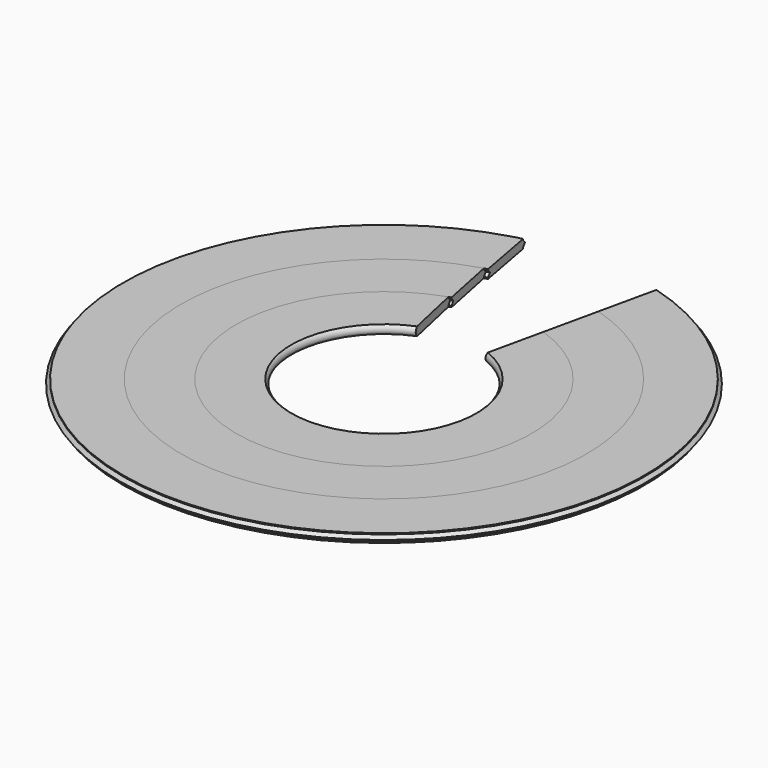
from build123d import *

# Parameters (mm, degrees)
F5_DEPTH = 1.5
F6_ANGLE = 1
F7_ANGLE = 2


with BuildPart() as f1:
    # F0 (on Front) → F1 (revolve)
    with BuildSketch(Plane.XZ):
        with BuildLine():
            Line((-16, 0.75), (-25.5, 0.75))
            Line((-25.5, 0.75), (-25.5, 0.55))
            Line((-25.5, 0.55), (-26.05, 0))
            Line((-26.05, 0), (-25.5, -0.55))
            Line((-25.5, -0.55), (-25.5, -0.75))
            Line((-25.5, -0.75), (-16, -0.75))
            ThreePointArc((-16, -0.75), (-15.5986121811, 0), (-16, 0.75))
        make_face()
        Polygon((-25.5, 0.75), (-26, 0.75), (-26, 0.55), (-26.55, 0), (-26, -0.55), (-26, -0.75), (-25.5, -0.75), (-25.5, -0.55), (-26.05, 0), (-25.5, 0.55), align=None)
    revolve(axis=Axis((0, 0, 8.4824059159), (0, 0, 1)))


with BuildPart() as f2:
    # F0 (on Front) → F2 (revolve)
    with BuildSketch(Plane.XZ):
        Polygon((-26, 0.75), (-35, 0.75), (-35, 0.55), (-35.55, 0), (-35, -0.55), (-35, -0.75), (-26, -0.75), (-26, -0.55), (-26.55, 0), (-26, 0.55), align=None)
        Polygon((-25.5, 0.75), (-26, 0.75), (-26, 0.55), (-26.55, 0), (-26, -0.55), (-26, -0.75), (-25.5, -0.75), (-25.5, -0.55), (-26.05, 0), (-25.5, 0.55), align=None)
        Polygon((-35, 0.75), (-35.5, 0.75), (-35.5, 0.55), (-36.05, 0), (-35.5, -0.55), (-35.5, -0.75), (-35, -0.75), (-35, -0.55), (-35.55, 0), (-35, 0.55), align=None)
    revolve(axis=Axis((0, 0, 8.4824059159), (0, 0, 1)))


with BuildPart() as f3:
    # F0 (on Front) → F3 (revolve)
    with BuildSketch(Plane.XZ):
        Polygon((-35.5, 0.75), (-45, 0.75), (-45, 0.55), (-45.55, 0), (-45, -0.55), (-45, -0.75), (-35.5, -0.75), (-35.5, -0.55), (-36.05, 0), (-35.5, 0.55), align=None)
        Polygon((-35, 0.75), (-35.5, 0.75), (-35.5, 0.55), (-36.05, 0), (-35.5, -0.55), (-35.5, -0.75), (-35, -0.75), (-35, -0.55), (-35.55, 0), (-35, 0.55), align=None)
    revolve(axis=Axis((0, 0, 8.4824059159), (0, 0, 1)))


with BuildPart() as f5_tool:
    # F4 (on face) → F5 (new body, through all)
    with BuildSketch(Plane.XY.offset(0.75)):
        with BuildLine():
            Line((-8.2945057155, 24.6414523707), (-6.1099268561, 14.7874539327))
            ThreePointArc((-6.1099268561, 14.7874539327), (0, 16), (6.1099268561, 14.7874539327))
            Line((6.1099268561, 14.7874539327), (8.2945057155, 24.6414523707))
            ThreePointArc((8.2945057155, 24.6414523707), (0, 26), (-8.2945057155, 24.6414523707))
        make_face()
        with BuildLine():
            Line((-6.1099268561, 14.7874539327), (-6, 14.291605928))
            ThreePointArc((-6, 14.291605928), (0, 15.5), (6, 14.291605928))
            Line((6, 14.291605928), (6.1099268561, 14.7874539327))
            ThreePointArc((6.1099268561, 14.7874539327), (0, 16), (-6.1099268561, 14.7874539327))
        make_face()
        with BuildLine():
            Line((-12.5396268012, 43.7899561508), (-8.2945057155, 24.6414523707))
            ThreePointArc((-8.2945057155, 24.6414523707), (0, 26), (8.2945057155, 24.6414523707))
            Line((8.2945057155, 24.6414523707), (12.5396268012, 43.7899561508))
            ThreePointArc((12.5396268012, 43.7899561508), (0, 45.55), (-12.5396268012, 43.7899561508))
        make_face()
    extrude(amount=-F5_DEPTH)


with BuildPart() as f1_1:
    add(f1.part)

    # F5: cut by f5_tool
    add(f5_tool.part, mode=Mode.SUBTRACT)


with BuildPart() as f2_1:
    add(f2.part)

    # F5: cut by f5_tool
    add(f5_tool.part, mode=Mode.SUBTRACT)

    # F5_face (on face) → F6 (revolve)
    with BuildSketch(Plane(origin=(-9.3162931707, 29.2504377339, 0), x_dir=(-0.2164396139, 0.9762960071, 0), z_dir=(0.9762960071, 0.2164396139, 0))):
        with BuildLine():
            Line((4.8186950678, 0.75), (-5.223796234, 0.75))
            Line((-5.223796234, 0.75), (-5.223796234, 0.55))
            add(Edge.make_bspline(
                [(-4.6706047852, 0), (-4.9501515794, 0.2779681938), (-5.223796234, 0.55)],
                knots=[-2.9334753636, -2.9334753636, -2.9334753636, -2.9120122138, -2.9120122138, -2.9120122138], degree=2, weights=[1, 1.0000575839, 1]))
            add(Edge.make_bspline(
                [(-5.223796234, -0.55), (-4.9501515794, -0.2779681938), (-4.6706047852, 0)],
                knots=[2.9120122138, 2.9120122138, 2.9120122138, 2.9334753636, 2.9334753636, 2.9334753636], degree=2, weights=[1, 1.0000575839, 1]))
            Line((-5.223796234, -0.55), (-5.223796234, -0.75))
            Line((-5.223796234, -0.75), (4.8186950678, -0.75))
            Line((4.8186950678, -0.75), (4.8186950678, -0.55))
            add(Edge.make_bspline(
                [(4.8186950678, -0.55), (5.092399633, -0.2771266059), (5.3703446915, 0)],
                knots=[3.2442982582, 3.2442982582, 3.2442982582, 3.2597185393, 3.2597185393, 3.2597185393], degree=2, weights=[1, 1.0000297233, 1]))
            add(Edge.make_bspline(
                [(5.3703446915, 0), (5.092399633, 0.2771266059), (4.8186950678, 0.55)],
                knots=[-3.2597185393, -3.2597185393, -3.2597185393, -3.2442982582, -3.2442982582, -3.2442982582], degree=2, weights=[1, 1.0000297233, 1]))
            Line((4.8186950678, 0.55), (4.8186950678, 0.75))
        make_face()
    revolve(axis=Axis((0, 0, 8.4824059159), (0, 0, -1)), revolution_arc=F6_ANGLE)


with BuildPart() as f3_1:
    add(f3.part)

    # F5: cut by f5_tool
    add(f5_tool.part, mode=Mode.SUBTRACT)

    # F5_face (on face) → F7 (revolve)
    with BuildSketch(Plane(origin=(-9.3162931707, 29.2504377339, 0), x_dir=(-0.2164396139, 0.9762960071, 0), z_dir=(0.9762960071, 0.2164396139, 0))):
        with BuildLine():
            add(Edge.make_bspline(
                [(14.8925308624, 0), (14.6153432848, 0.2766765991), (14.3415026483, 0.55)],
                knots=[-3.4941735673, -3.4941735673, -3.4941735673, -3.4820027221, -3.4820027221, -3.4820027221], degree=2, weights=[1, 1.0000185162, 1]))
            Line((14.3415026483, 0.55), (14.3415026483, 0.75))
            Line((14.3415026483, 0.75), (4.3171502115, 0.75))
            Line((4.3171502115, 0.75), (4.3171502115, 0.55))
            add(Edge.make_bspline(
                [(4.8688471524, 0), (4.5908481978, 0.2771571192), (4.3171502115, 0.55)],
                knots=[-3.245709999, -3.245709999, -3.245709999, -3.2300697953, -3.2300697953, -3.2300697953], degree=2, weights=[1, 1.0000305772, 1]))
            add(Edge.make_bspline(
                [(4.3171502115, -0.55), (4.5908481978, -0.2771571192), (4.8688471524, 0)],
                knots=[3.2300697953, 3.2300697953, 3.2300697953, 3.245709999, 3.245709999, 3.245709999], degree=2, weights=[1, 1.0000305772, 1]))
            Line((4.3171502115, -0.55), (4.3171502115, -0.75))
            Line((4.3171502115, -0.75), (14.3415026483, -0.75))
            Line((14.3415026483, -0.75), (14.3415026483, -0.55))
            add(Edge.make_bspline(
                [(14.3415026483, -0.55), (14.6153432848, -0.2766765991), (14.8925308624, 0)],
                knots=[3.4820027221, 3.4820027221, 3.4820027221, 3.4941735673, 3.4941735673, 3.4941735673], degree=2, weights=[1, 1.0000185162, 1]))
        make_face()
    revolve(axis=Axis((0, 0, 8.4824059159), (0, 0, -1)), revolution_arc=F7_ANGLE)


solid = Compound([f1_1.part, f2_1.part, f3_1.part])
